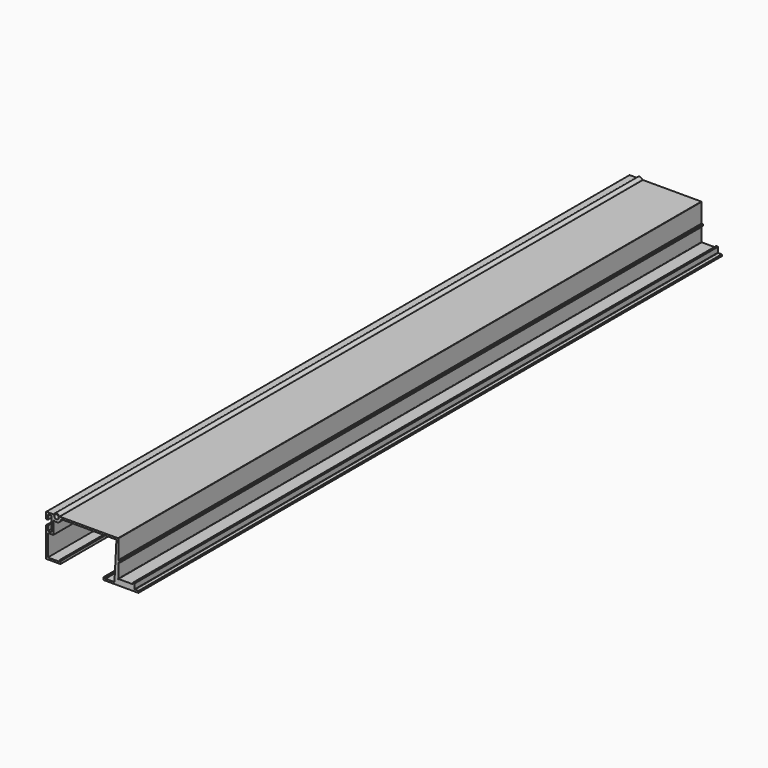
from build123d import *

# Parameters (mm, degrees)
F1_DEPTH = 1000
F2_R     = 0.5
F4_DEPTH = 1000
F5_W     = 2
F5_H     = 2.5
F5_W_2   = 2.4
F5_H_2   = 2
F6_DEPTH = 1000
F7_R     = 0.5
F8_R     = 3
F9_DEPTH = 1000


# Not quite as in the source:
# - a feature names something its author has since deleted; it is built from what else it names


with BuildPart() as f1:
    # F0 (on Front) → F1 (new body)
    with BuildSketch(Plane.XZ):
        with BuildLine():
            Line((-33, 57), (-113.9880191388, 57))
            ThreePointArc((-113.9880191388, 57), (-117.75, 51.45), (-121.5119808612, 57))
            Line((-121.5119808612, 57), (-132, 57))
            Line((-132, 57), (-132, 48))
            Line((-132, 48), (-129.5, 48))
            Line((-129.5, 48), (-129.5, 54.5))
            Line((-129.5, 54.5), (-124.3, 54.5))
            Line((-124.3, 54.5), (-124.3, 34.5))
            Line((-124.3, 34.5), (-129.5, 34.5))
            Line((-129.5, 34.5), (-129.5, 41))
            Line((-129.5, 41), (-132, 41))
            Line((-132, 41), (-132, 0))
            Line((-132, 0), (-112, 0))
            Line((-112, 0), (-112, 4))
            Line((-112, 4), (-114.5, 4))
            Line((-114.5, 4), (-114.5, 2.5))
            Line((-114.5, 2.5), (-129.5, 2.5))
            Line((-129.5, 2.5), (-129.5, 32))
            Line((-129.5, 32), (-121.8, 32))
            Line((-121.8, 32), (-121.8, 50.3521849295))
            ThreePointArc((-121.8, 50.3521849295), (-115.3481082383, 49.4062806132), (-111.2767859606, 54.5))
            Line((-111.2767859606, 54.5), (-35.5, 54.5))
            Line((-35.5, 54.5), (-38.2252045227, 2.5))
            Line((-38.2252045227, 2.5), (-50.5, 2.5))
            Line((-50.5, 2.5), (-50.5, 4))
            Line((-50.5, 4), (-53, 4))
            Line((-53, 4), (-53, 0))
            Line((-53, 0), (-5, 0))
            Line((-5, 0), (-5, 2.5))
            Line((-5, 2.5), (-10.5, 2.5))
            Line((-10.5, 2.5), (-10.5, 8))
            Line((-10.5, 8), (-33, 8))
            Line((-33, 8), (-33, 57))
        make_face()
    extrude(amount=F1_DEPTH)

    # F2
    f2_edges = [f1.edges().sort_by_distance(p)[0] for p in [
        (-132, -500, 57),
        (-132, -500, 41),
        (-112, -500, 0),
        (-33, -500, 57),
        (-121.511981, -500, 57),
        (-113.988019, -500, 57),
        (-132, -500, 48),
        (-114.5, -500, 4),
        (-112, -500, 4),
        (-53, -500, 4),
        (-50.5, -500, 4),
        (-53, -500, 0),
        (-132, -500, 0),
        (-121.8, -500, 32),
        (-38.225205, -500, 2.5),
        (-35.5, -500, 54.5),
        (-111.276786, -500, 54.5),
        (-121.8, -500, 50.352185),
        (-5, -500, 0),
        (-5, -500, 2.5),
        (-10.5, -500, 2.5),
    ]]
    fillet(f2_edges, radius=F2_R)

    # F3 (on face) → F4 (cut)
    with BuildSketch(Plane.XZ.offset(1000)):
        with BuildLine():
            ThreePointArc((-33, 8.5), (-33.3535533906, 7.6464466094), (-32.5, 8))
            Line((-32.5, 8), (-33, 8))
            Line((-33, 8), (-33, 8.5))
        make_face()
    extrude(amount=-F4_DEPTH, mode=Mode.SUBTRACT)

    # F5 (on face) → F6 (join)
    with BuildSketch(Plane.XZ.offset(1000)):
        with Locations((-32, 29.35)):
            Rectangle(F5_W, F5_H)
        with Locations((-11.7, 9)):
            Rectangle(F5_W_2, F5_H_2)
    extrude(amount=-F6_DEPTH)

    # F7
    f7_edges = [f1.edges().sort_by_distance(p)[0] for p in [
        (-31, -500, 30.6),
        (-10.5, -500, 10),
    ]]
    fillet(f7_edges, radius=F7_R)


with BuildPart() as f9:
    # F8 (on face) → F9 (new body)
    with BuildSketch(Plane.XZ.offset(1000)):
        with BuildLine():
            ThreePointArc((-121.7009751181, 56.3901098901), (-118.1978006096, 51.4748323496), (-113.7, 55.5))
            ThreePointArc((-113.7, 55.5), (-113.7248323496, 55.9478006096), (-113.7990248819, 56.3901098901))
            ThreePointArc((-113.7990248819, 56.3901098901), (-117.75, 59.55), (-121.7009751181, 56.3901098901))
        make_face()
        with Locations((-117.75, 55.5)):
            Circle(F8_R, mode=Mode.SUBTRACT)
    extrude(amount=-F9_DEPTH)


solid = Compound([f1.part, f9.part])
